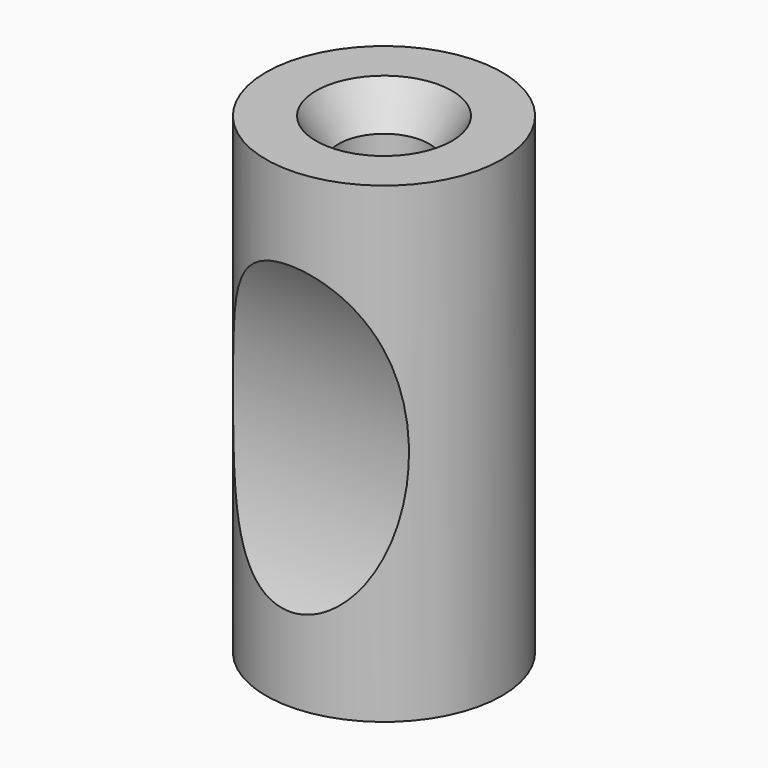
from build123d import *

# Parameters (mm, degrees)
F0_R          = 1.15
F0_R_2        = 0.4
F1_DEPTH      = 6
F0_R_3        = 3
F2_DEPTH      = 12
F3_SIZE2      = 0.5773502692
F3_SIZE       = 1
F4_R          = 8
F5_DEPTH      = 25
F5_DEPTH_BACK = 25


with BuildPart() as f1:
    # F0 (on Top) → F1 (new body)
    with BuildSketch(Plane.XY):
        Circle(F0_R)
        Circle(F0_R_2, mode=Mode.SUBTRACT)
    extrude(amount=F1_DEPTH)

    # F0 (on Top) → F2 (join)
    with BuildSketch(Plane.XY):
        Circle(F0_R_3)
        Circle(F0_R, mode=Mode.SUBTRACT)
    extrude(amount=F2_DEPTH)

    # F3
    f3_edges = [f1.edges().sort_by_distance(p)[0] for p in [
        (-1.15, 0, 12),
    ]]
    f3_side = f1.faces().sort_by_distance((-1.15, 0, 9))[0]
    chamfer(f3_edges, length=F3_SIZE, length2=F3_SIZE2, reference=f3_side)

    # F4 (on Right) → F5 (cut, two sides)
    with BuildSketch(Plane.YZ) as f5_sk:
        with Locations((10, 6)):
            Circle(F4_R)
        with Locations((-10, 6)):
            Circle(F4_R)
    extrude(amount=-F5_DEPTH, mode=Mode.SUBTRACT)
    extrude(f5_sk.sketch, amount=F5_DEPTH_BACK, mode=Mode.SUBTRACT)


solid = f1.part
